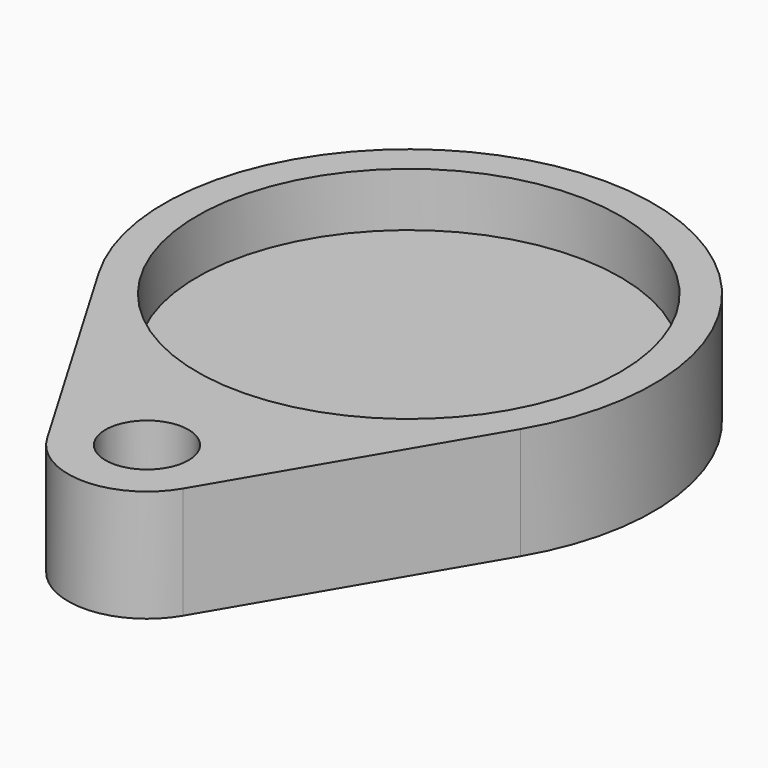
from build123d import *

# Parameters (mm, degrees)
F0_R      = 10
F1_DEPTH  = 1
F2_R      = 11.8
F3_DEPTH  = 1
F4_R      = 11.8
F4_R_2    = 10
F5_DEPTH  = 1
F6_R      = 11.8
F7_DEPTH  = 3.4
F8_R      = 10.2
F9_DEPTH  = 2.6
F10_R     = 2
F11_DEPTH = 5.4


with BuildPart() as f1:
    # F0 (on Top) → F1 (new body)
    with BuildSketch(Plane.XY):
        Circle(F0_R)
    extrude(amount=F1_DEPTH)


with BuildPart() as f3:
    # F2 (on face) → F3 (new body)
    with BuildSketch(Plane(origin=(0, 0, 0), x_dir=(1, 0, 0), z_dir=(0, 0, -1))):
        Circle(F2_R)
    extrude(amount=F3_DEPTH)

    # F4 (on face) → F5 (join)
    with BuildSketch(Plane.XY):
        Circle(F4_R)
        Circle(F4_R_2, mode=Mode.SUBTRACT)
    extrude(amount=F5_DEPTH)

    # F6 (on face) → F7 (join)
    with BuildSketch(Plane.XY.offset(1)):
        Circle(F6_R)
    extrude(amount=F7_DEPTH)

    # F8 (on face) → F9 (cut)
    with BuildSketch(Plane.XY.offset(4.4)):
        Circle(F8_R)
    extrude(amount=-F9_DEPTH, mode=Mode.SUBTRACT)

    # F10 (on face) → F11 (join, through all)
    with BuildSketch(Plane(origin=(0, 0, -1), x_dir=(1, 0, 0), z_dir=(0, 0, -1))):
        with BuildLine():
            ThreePointArc((-3.2754372895, 17.7062096148), (-0.9983331858, 12.113166694), (3.8, 15.7796815038))
            ThreePointArc((3.8, 15.7796815038), (3.6665148097, 16.7780146896), (3.2754372895, 17.7062096148))
            ThreePointArc((3.2754372895, 17.7062096148), (0, 19.5796815038), (-3.2754372895, 17.7062096148))
        make_face()
        with Locations((0, 15.7796815038)):
            Circle(F10_R, mode=Mode.SUBTRACT)
        with BuildLine():
            ThreePointArc((3.2754372895, 17.7062096148), (3.6665148097, 16.7780146896), (3.8, 15.7796815038))
            ThreePointArc((3.8, 15.7796815038), (-0.9983331858, 12.113166694), (-3.2754372895, 17.7062096148))
            Line((-3.2754372895, 17.7062096148), (-10.1710947411, 5.9823767658))
            ThreePointArc((-10.1710947411, 5.9823767658), (0, 11.8), (10.1710947411, 5.9823767658))
            Line((10.1710947411, 5.9823767658), (3.2754372895, 17.7062096148))
        make_face()
    extrude(amount=-F11_DEPTH)


solid = Compound([f1.part, f3.part])
